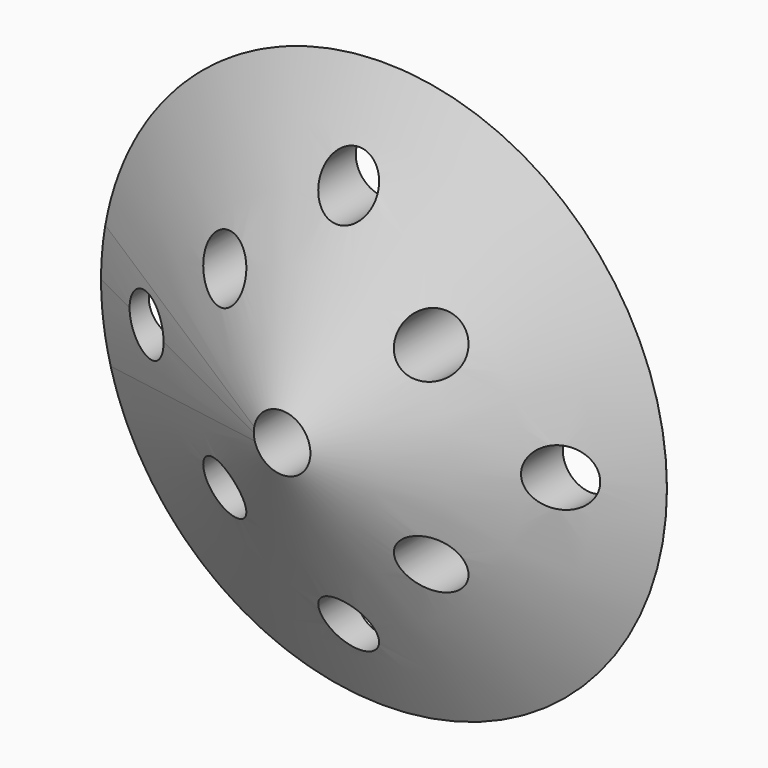
from build123d import *
from build123d import SkipClean  # not in build123d's __all__

# Parameters (mm, degrees)
F0_R     = 50.8
F1_DEPTH = 25.4
F4_ANGLE = 350
F5_ANGLE = 25
F7_R     = 5.08
F8_DEPTH = 25.401


with BuildPart() as f1:
    # F0 (on Front) → F1 (new body)
    with BuildSketch(Plane.XZ):
        Circle(F0_R)
    extrude(amount=F1_DEPTH)

    # F3 (on Top) → F4 (revolve, cut)
    with BuildSketch(Plane.XY):
        Polygon((-50.8231706917, -25.4051908851), (-0.0053378481, -25.4051908851), (-50.8231706917, 0), align=None)
    revolve(axis=Axis((0, -21.8290705234, 0), (0, -1, 0)), revolution_arc=F4_ANGLE, mode=Mode.SUBTRACT)

    # F4_face (on face) → F5 (revolve, cut)
    with BuildSketch(Plane(origin=(-33.3573166691, -16.9371945491, 5.8817949328), x_dir=(1, 0, 0), z_dir=(0.1736481777, 0, 0.984807753))):
        Polygon((-16.9280929531, -8.4628054509), (33.8561859063, -8.4628054509), (-16.9280929531, 16.9256109019), align=None)
    with SkipClean():  # cleaning this boolean's faces spoils the solid; the shape is the same uncleaned
        revolve(axis=Axis((0, -21.8290705234, 0), (0, -1, 0)), revolution_arc=F5_ANGLE, mode=Mode.SUBTRACT)

    # F7 (on offset) → F8 (cut, through all)
    with BuildSketch(Plane.XZ.offset(25.4)):
        with Locations((0, -34.6310168025)):
            Circle(F7_R)
        with Locations((0, 34.6310168025)):
            Circle(F7_R)
        with Locations((-37.1662841191, 0)):
            Circle(F7_R)
        with Locations((37.1662841191, 0)):
            Circle(F7_R)
        Circle(F7_R)
        with Locations((-18.5831420596, -17.3155084013)):
            Circle(F7_R)
        with Locations((-18.5831420596, 17.3155084013)):
            Circle(F7_R)
        with Locations((18.5831420596, 17.3155084013)):
            Circle(F7_R)
        with Locations((18.5831420596, -17.3155084013)):
            Circle(F7_R)
    with SkipClean():  # cleaning this boolean's faces spoils the solid; the shape is the same uncleaned
        extrude(amount=-F8_DEPTH, mode=Mode.SUBTRACT)


solid = f1.part
